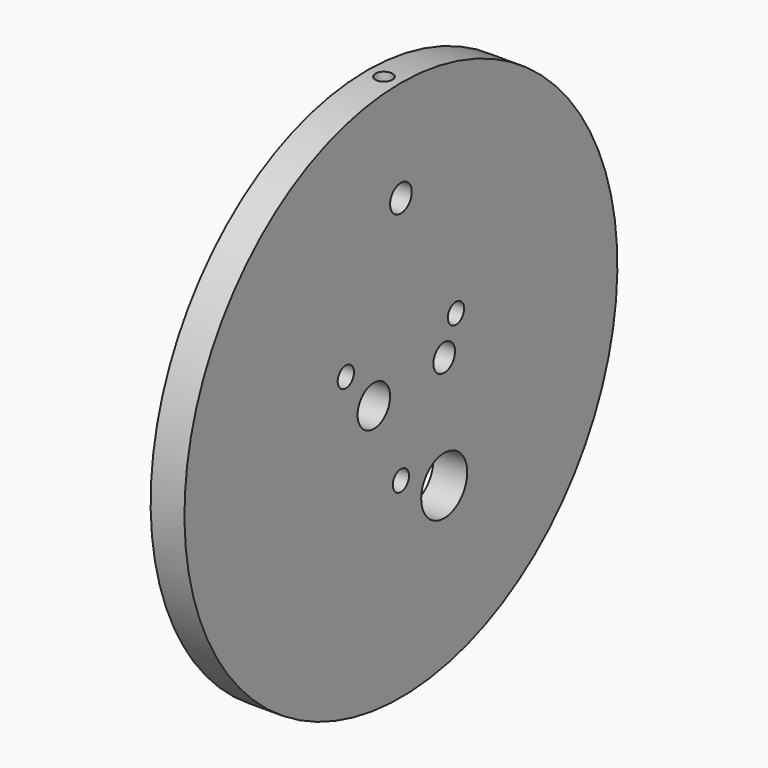
from build123d import *

# Parameters (mm, degrees)
F0_W            = 5
F0_H            = 40
F3_D            = 4
F4_D            = 4
F5_D            = 6
F6_D            = 8.5
F8_D            = 3
F8_CSINK_D      = 6
F8_CSINK_ANGLE  = 90
F8_COPIES_COUNT = 3
F11_D           = 2.5
F11_DEPTH       = 14.6
F11_START       = 0.0195361
F11_TIP         = 0.7510757738


# Not quite as in the source:
# - a pattern or mirror of a feature is missing from the dataset's text; its kind, count and spacing are read off the source's solid


with BuildPart() as f1:
    # F0 (on Front) → F1 (revolve)
    with BuildSketch(Plane.XZ):
        with Locations((2.5, 20)):
            Rectangle(F0_W, F0_H)
    revolve(axis=Axis((2.5, 0, 0), (-1, 0, 0)))

    # F3 (through all)
    with Locations(Plane.YZ.offset(5)):
        with Locations((8, 1)):
            Hole(F3_D / 2)

    # F4 (through all)
    with Locations(Plane.YZ.offset(5)):
        with Locations((0, 25)):
            Hole(F4_D / 2)

    # F5 (through all)
    with Locations(Plane.YZ.offset(5)):
        with Locations((-5, 0)):
            Hole(F5_D / 2)

    # F6 (through all)
    with Locations(Plane.YZ.offset(5)):
        with Locations((8, -15.6675087226)):
            Hole(F6_D / 2)

    # F8 (through all)
    with Locations(Plane(origin=(0, 0, 0), x_dir=(0, -1, 0), z_dir=(-1, 0, 0))):
        with Locations((0, -11.75)):
            f8 = CounterSinkHole(F8_D / 2, F8_CSINK_D / 2, counter_sink_angle=F8_CSINK_ANGLE)

    # F8_copies: F8 ×3 about axis
    f8_copies_axis = Axis((0, 0, 0), (1, 0, 0))
    for i in range(1, F8_COPIES_COUNT):
        add(f8.rotate(f8_copies_axis, i * 360 / F8_COPIES_COUNT), mode=Mode.SUBTRACT)

    # F11
    # its depths count from where the whole tool has entered the part; down to there all is cleared
    with Locations(Plane.XY.offset(40).offset(-F11_START)):
        with Locations((2.5, 0)):
            Hole(F11_D / 2, depth=F11_DEPTH)
            with Locations((0, 0, -(F11_DEPTH + F11_TIP / 2))):  # 118° drill point
                Cone(0, F11_D / 2, F11_TIP, mode=Mode.SUBTRACT)


solid = f1.part
